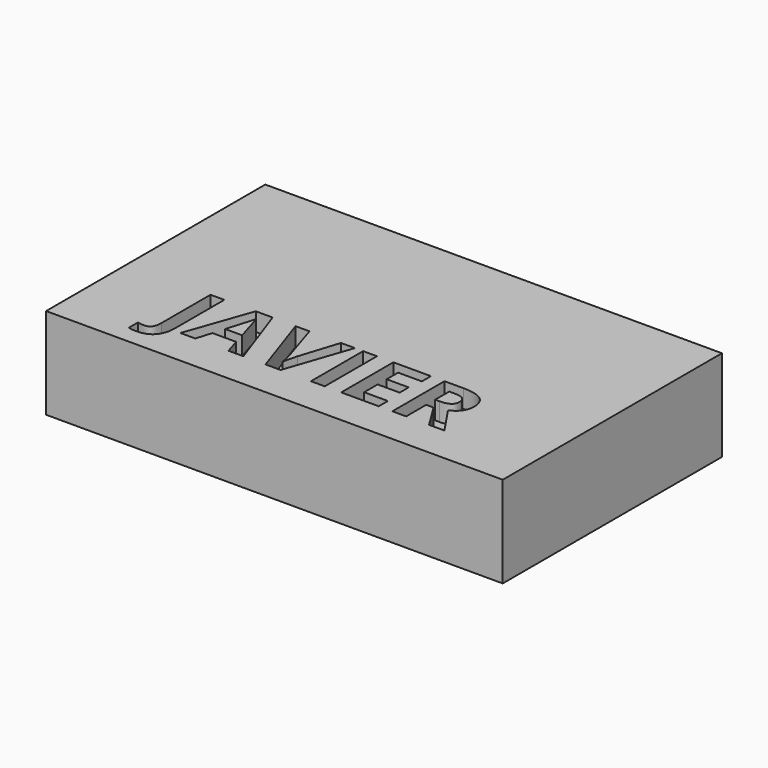
from build123d import *

# Parameters (mm, degrees)
F0_W         = 25
F0_H         = 15
F1_DEPTH     = 5
F2_TEXT_SIZE = 5
F3_DEPTH     = 1


# Not quite as in the source:
# - Text() gives the source's letters only with a copy of the font that has no kerning and outlines rounded to 1/6400 em; it was checked with that copy


with BuildPart() as f1:
    # F0 (on Top) → F1 (new body)
    with BuildSketch(Plane.XY):
        Rectangle(F0_W, F0_H)
    extrude(amount=F1_DEPTH)

    # F2 (on face) → F3 (cut)
    with BuildSketch(Plane.XY.offset(5)):
        with Locations((-8.403125, -5.5)):
            Text('JAVIER', F2_TEXT_SIZE, font='Open Sans', font_style=FontStyle.BOLD, text_align=(TextAlign.LEFT, TextAlign.BOTTOM))
    extrude(amount=-F3_DEPTH, mode=Mode.SUBTRACT)


solid = f1.part
